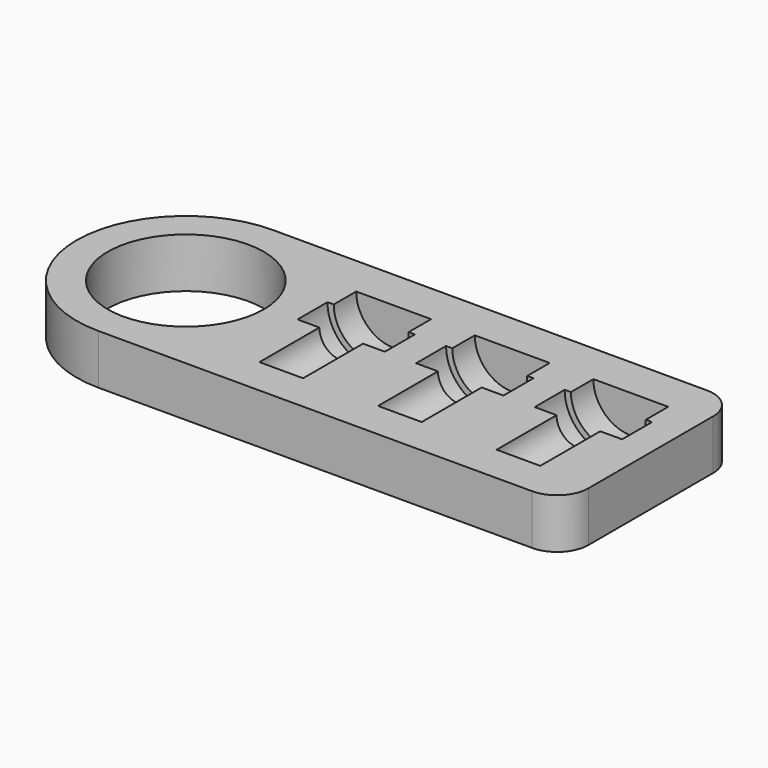
from build123d import *

# Parameters (mm, degrees)
F0_R         = 12.5
F1_DEPTH     = 8
F6_TEXT_SIZE = 5.5555555556
F7_DEPTH     = 1


# Not quite as in the source:
# - Text() gives the source's letters only with a copy of the font that has no kerning and outlines rounded to 1/6400 em; it was checked with that copy


with BuildPart() as f1:
    # F0 (on Top) → F1 (new body)
    with BuildSketch(Plane.XY):
        with BuildLine():
            ThreePointArc((0, 17.5), (5.1256313292, 5.1256313292), (17.5, 0))
            Line((17.5, 0), (87, 0))
            ThreePointArc((87, 0), (90.5355339059, 1.4644660941), (92, 5))
            Line((92, 5), (92, 30))
            ThreePointArc((92, 30), (90.5355339059, 33.5355339059), (87, 35))
            Line((87, 35), (17.5, 35))
            ThreePointArc((17.5, 35), (5.1256313292, 29.8743686708), (0, 17.5))
        make_face()
        with Locations((17.5, 17.5)):
            Circle(F0_R, mode=Mode.SUBTRACT)
    extrude(amount=F1_DEPTH)

    # F2 (on face) → F3 (revolve, cut)
    with BuildSketch(Plane.XY.offset(8)):
        Polygon((42, 18), (42, 6), (45.5, 6), (45.5, 18), (49, 18), (49, 24), (48, 24), (48, 28.5), (42, 28.5), (42, 24), align=None)
    revolve(axis=Axis((42, 12, 8), (0, 1, 0)), mode=Mode.SUBTRACT)

    # F2 (on face) → F4 (revolve, cut)
    with BuildSketch(Plane.XY.offset(8)):
        Polygon((61, 18), (61, 6), (64.5, 6), (64.5, 18), (68, 18), (68, 24), (67, 24), (67, 28.5), (61, 28.5), (61, 24), align=None)
    revolve(axis=Axis((61, 12, 8), (0, 1, 0)), mode=Mode.SUBTRACT)

    # F2 (on face) → F5 (revolve, cut)
    with BuildSketch(Plane.XY.offset(8)):
        Polygon((80, 18), (80, 6), (83.5, 6), (83.5, 18), (87, 18), (87, 24), (86, 24), (86, 28.5), (80, 28.5), (80, 24), align=None)
    revolve(axis=Axis((80, 12, 8), (0, 1, 0)), mode=Mode.SUBTRACT)

    # F6 (on face) → F7 (cut)
    with BuildSketch(Plane(origin=(0, 0, 0), x_dir=(1, 0, 0), z_dir=(0, 0, -1))):
        with Locations((30, -9)):
            Text('863, 793', F6_TEXT_SIZE, font='Open Sans', text_align=(TextAlign.LEFT, TextAlign.BOTTOM))
    extrude(amount=-F7_DEPTH, mode=Mode.SUBTRACT)


solid = f1.part
